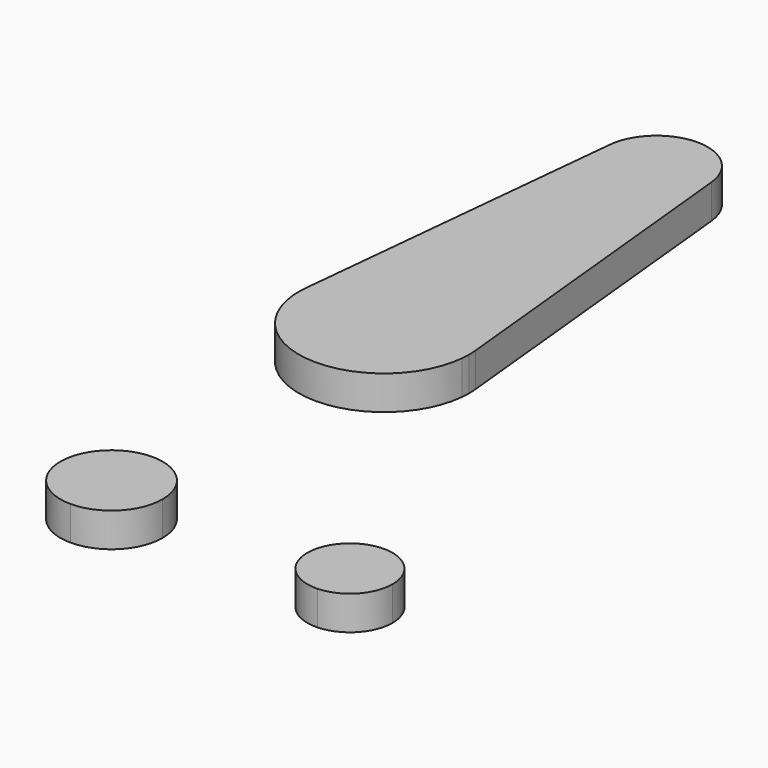
from build123d import *

# Parameters (mm, degrees)
F1_DEPTH = 0.25
F2_DEPTH = 0.25


with BuildPart() as f1:
    # F0 (on Top) → F1 (new body)
    with BuildSketch(Plane.XY):
        with BuildLine():
            ThreePointArc((-0.6218671482, 2.4375), (0, 1.875), (0.6218671482, 2.4375))
            ThreePointArc((0.6218671482, 2.4375), (0.6242162957, 2.4687107656), (0.625, 2.5))
            ThreePointArc((0.625, 2.5), (0.6242162957, 2.5312892344), (0.6218671482, 2.5625))
            ThreePointArc((0.6218671482, 2.5625), (0, 3.125), (-0.6218671482, 2.5625))
            ThreePointArc((-0.6218671482, 2.5625), (-0.625, 2.5), (-0.6218671482, 2.4375))
        make_face()
        with BuildLine():
            Line((-0.3731202889, 5.0375), (-0.6218671482, 2.5625))
            ThreePointArc((-0.6218671482, 2.5625), (0, 3.125), (0.6218671482, 2.5625))
            Line((0.6218671482, 2.5625), (0.3731202889, 5.0375))
            ThreePointArc((0.3731202889, 5.0375), (0.3745297774, 5.0187735406), (0.375, 5))
            ThreePointArc((0.375, 5), (-0.0187735406, 4.6254702226), (-0.3731202889, 5.0375))
        make_face()
        with BuildLine():
            ThreePointArc((0.3731202889, 5.0375), (0, 5.375), (-0.3731202889, 5.0375))
            ThreePointArc((-0.3731202889, 5.0375), (-0.0187735406, 4.6254702226), (0.375, 5))
            ThreePointArc((0.375, 5), (0.3745297774, 5.0187735406), (0.3731202889, 5.0375))
        make_face()
    extrude(amount=F1_DEPTH)


with BuildPart() as f1b:
    # F0 (on Top) → F1, piece 2 (new body)
    with BuildSketch(Plane.XY):
        with BuildLine():
            ThreePointArc((1.7611607143, 0.3123006379), (1.4375000007, 2.12117e-05), (1.7611183179, -0.3123021502))
            ThreePointArc((1.7611183179, -0.3123021502), (1.9748674324, -0.2170043498), (2.0625, 0))
            ThreePointArc((2.0625, 0), (1.9748821616, 0.2169890859), (1.7611607143, 0.3123006379))
        make_face()
    extrude(amount=F1_DEPTH)


with BuildPart() as f1c:
    # F0 (on Top) → F1, piece 3 (new body)
    with BuildSketch(Plane.XY):
        with BuildLine():
            ThreePointArc((0, -0.375), (0.2651650429, -0.2651650429), (0.375, 0))
            ThreePointArc((0.375, 0), (-0.2651650429, 0.2651650429), (0, -0.375))
        make_face()
    extrude(amount=F1_DEPTH)


with BuildPart() as f2:
    # F0 (on Top) → F2 (new body)
    with BuildSketch(Plane.XY):
        with BuildLine():
            ThreePointArc((-0.6218671482, 2.4375), (0, 1.875), (0.6218671482, 2.4375))
            ThreePointArc((0.6218671482, 2.4375), (0.6242162957, 2.4687107656), (0.625, 2.5))
            ThreePointArc((0.625, 2.5), (0.6242162957, 2.5312892344), (0.6218671482, 2.5625))
            ThreePointArc((0.6218671482, 2.5625), (0, 3.125), (-0.6218671482, 2.5625))
            ThreePointArc((-0.6218671482, 2.5625), (-0.625, 2.5), (-0.6218671482, 2.4375))
        make_face()
        with BuildLine():
            Line((-0.3731202889, 5.0375), (-0.6218671482, 2.5625))
            ThreePointArc((-0.6218671482, 2.5625), (0, 3.125), (0.6218671482, 2.5625))
            Line((0.6218671482, 2.5625), (0.3731202889, 5.0375))
            ThreePointArc((0.3731202889, 5.0375), (0.3745297774, 5.0187735406), (0.375, 5))
            ThreePointArc((0.375, 5), (-0.0187735406, 4.6254702226), (-0.3731202889, 5.0375))
        make_face()
        with BuildLine():
            ThreePointArc((0.3731202889, 5.0375), (0, 5.375), (-0.3731202889, 5.0375))
            ThreePointArc((-0.3731202889, 5.0375), (-0.0187735406, 4.6254702226), (0.375, 5))
            ThreePointArc((0.375, 5), (0.3745297774, 5.0187735406), (0.3731202889, 5.0375))
        make_face()
    extrude(amount=F2_DEPTH)


with BuildPart() as f2b:
    # F0 (on Top) → F2, piece 2 (new body)
    with BuildSketch(Plane.XY):
        with BuildLine():
            ThreePointArc((1.7611607143, 0.3123006379), (1.4375000007, 2.12117e-05), (1.7611183179, -0.3123021502))
            ThreePointArc((1.7611183179, -0.3123021502), (1.9748674324, -0.2170043498), (2.0625, 0))
            ThreePointArc((2.0625, 0), (1.9748821616, 0.2169890859), (1.7611607143, 0.3123006379))
        make_face()
    extrude(amount=F2_DEPTH)


with BuildPart() as f2c:
    # F0 (on Top) → F2, piece 3 (new body)
    with BuildSketch(Plane.XY):
        with BuildLine():
            ThreePointArc((0, -0.375), (0.2651650429, -0.2651650429), (0.375, 0))
            ThreePointArc((0.375, 0), (-0.2651650429, 0.2651650429), (0, -0.375))
        make_face()
    extrude(amount=F2_DEPTH)


solid = Compound([f1.part, f1b.part, f1c.part, f2.part, f2b.part, f2c.part])
